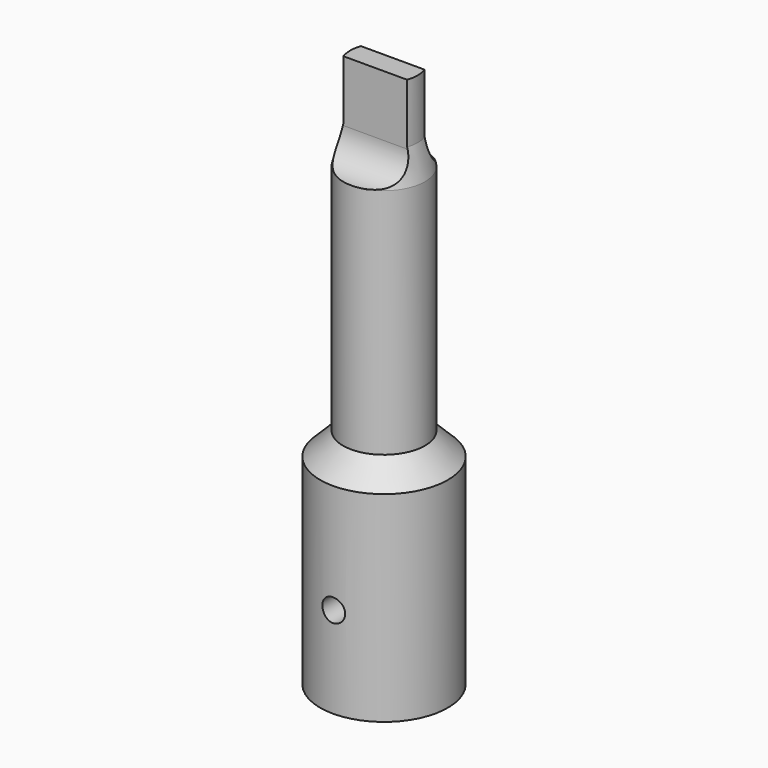
from build123d import *

# Parameters (mm, degrees)
F3_D     = 8
F3_DEPTH = 21.6
F3_TIP   = 2.403442
F4_W     = 2.2
F4_H     = 22
F5_DEPTH = 7.001
F7_D     = 2.5
F7_DEPTH = 7.001
F9_DEPTH = 12.5


with BuildPart() as f1:
    # F0 (on Front) → F1 (revolve)
    with BuildSketch(Plane.XZ):
        Polygon((0, 60), (0, 0), (7, 0), (7, 22), (4.5, 24.5), (4.5, 50), (3.7, 53.5), (3.7, 60), align=None)
    revolve(axis=Axis((0, 0, 41.622236), (0, 0, 1)))

    # F3
    with Locations(Plane(origin=(0, 0, 0), x_dir=(1, 0, 0), z_dir=(0, 0, -1))):
        with Locations((0, 0)):
            Hole(F3_D / 2, depth=F3_DEPTH)
            with Locations((0, 0, -(F3_DEPTH + F3_TIP / 2))):  # 118° drill point
                Cone(0, F3_D / 2, F3_TIP, mode=Mode.SUBTRACT)

    # F4 (on Front) → F5 (cut, through all)
    with BuildSketch(Plane.XZ):
        with Locations((0, 11)):
            Rectangle(F4_W, F4_H)
    extrude(amount=-F5_DEPTH, mode=Mode.SUBTRACT)

    # F7 (through all, one way)
    with BuildSketch(Plane(origin=(0, 0, 0), x_dir=(1, 0, 0), z_dir=(0, 1, 0))):
        with Locations((0, -10)):
            Circle(F7_D / 2)
    extrude(amount=-F7_DEPTH, mode=Mode.SUBTRACT)

    # F8 (on Right) → F9 (cut, symmetric)
    with BuildSketch(Plane.YZ):
        with BuildLine():
            Line((-1.2, 53.3), (-1.2, 60))
            Line((-1.2, 60), (-6.913031, 60))
            Line((-6.913031, 60), (-6.913031, 50))
            Line((-6.913031, 50), (-4.5, 50))
            ThreePointArc((-4.5, 50), (-2.166548, 50.966548), (-1.2, 53.3))
        make_face()
        with BuildLine():
            Line((6.913031, 60), (1.2, 60))
            Line((1.2, 60), (1.2, 53.3))
            ThreePointArc((1.2, 53.3), (2.166548, 50.966548), (4.5, 50))
            Line((4.5, 50), (6.913031, 50))
            Line((6.913031, 50), (6.913031, 60))
        make_face()
    extrude(amount=F9_DEPTH, both=True, mode=Mode.SUBTRACT)


solid = f1.part
